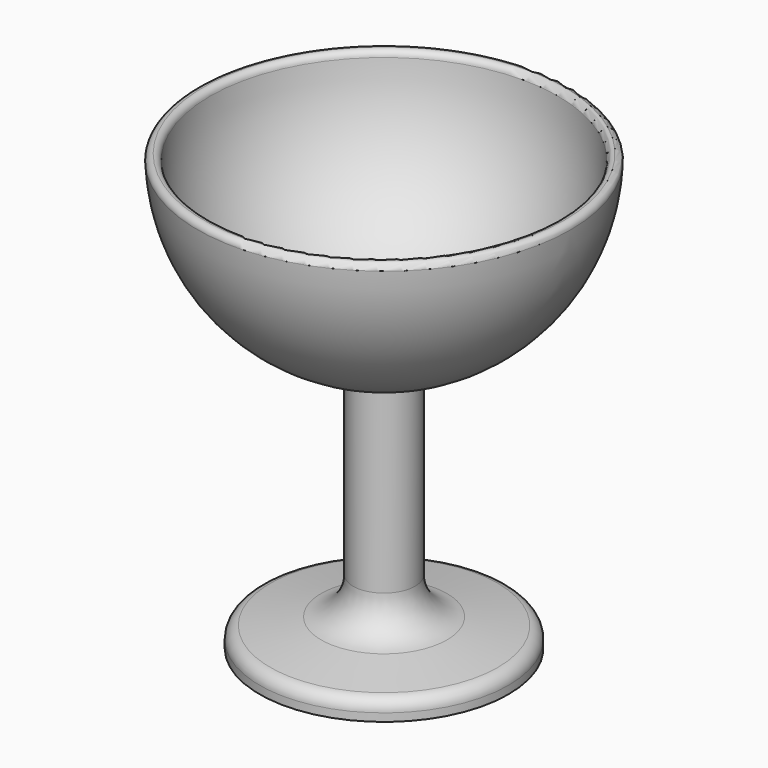
from build123d import *


# Not quite as in the source:
# - a fillet or chamfer that OpenCascade refuses, or shapes differently, is made with other operations: its cross-section is extruded or revolved along the edge and cut away or added


with BuildPart() as f1:
    # F0 (on Front) → F1 (revolve)
    with BuildSketch(Plane.XZ):
        with BuildLine():
            Line((0, 21), (0, 1.5))
            Line((0, 1.5), (8.5069227294, 0))
            Line((8.5069227294, 0), (10, 0))
            Line((10, 0), (10, 0.638732829))
            ThreePointArc((10, 0.638732829), (9.7577103301, 1.2913238615), (9.1482498888, 1.6276827623))
            Line((9.1482498888, 1.6276827623), (5.0552503337, 2.2412494438))
            ThreePointArc((5.0552503337, 2.2412494438), (3.2268690096, 3.2503261462), (2.5, 5.2080992435))
            Line((2.5, 5.2080992435), (2.5, 19.387505004))
            ThreePointArc((2.5, 19.387505004), (2.7193752502, 20.012505004), (3.28125, 20.3632859413))
            ThreePointArc((3.28125, 20.3632859413), (11.709371247, 25.625), (15, 35))
            Line((15, 35), (14, 35))
            ThreePointArc((14, 35), (9.8994949366, 25.1005050634), (0, 21))
        make_face()
    revolve(axis=Axis((0, 0, 19.0814351663), (0, 0, 1)))

    # F2: fillet of radius 0.5 on 2 edges, made by hand

    # F2_s1 → F2_t2 (revolve, cut)
    with BuildSketch(Plane.XZ):
        with BuildLine():
            ThreePointArc((14.4913767462, 35), (14.1439725793, 34.8595974761), (13.9916740998, 34.5172413793))
            ThreePointArc((13.9916740998, 34.5172413793), (13.9979183702, 34.7585847941), (14, 35))
            Line((14, 35), (14.4913767462, 35))
        make_face()
    revolve(axis=Axis((0, 0, 35), (0, 0, 1)), mode=Mode.SUBTRACT)

    # F2_s3 → F2_t4 (revolve, cut)
    with BuildSketch(Plane.XZ):
        with BuildLine():
            ThreePointArc((14.4913767462, 35), (14.8509742223, 34.8474041669), (14.9910793926, 34.4827586207))
            ThreePointArc((14.9910793926, 34.4827586207), (14.9977696823, 34.7413408509), (15, 35))
            Line((15, 35), (14.4913767462, 35))
        make_face()
    revolve(axis=Axis((0, 0, 35), (0, 0, 1)), mode=Mode.SUBTRACT)


solid = f1.part
